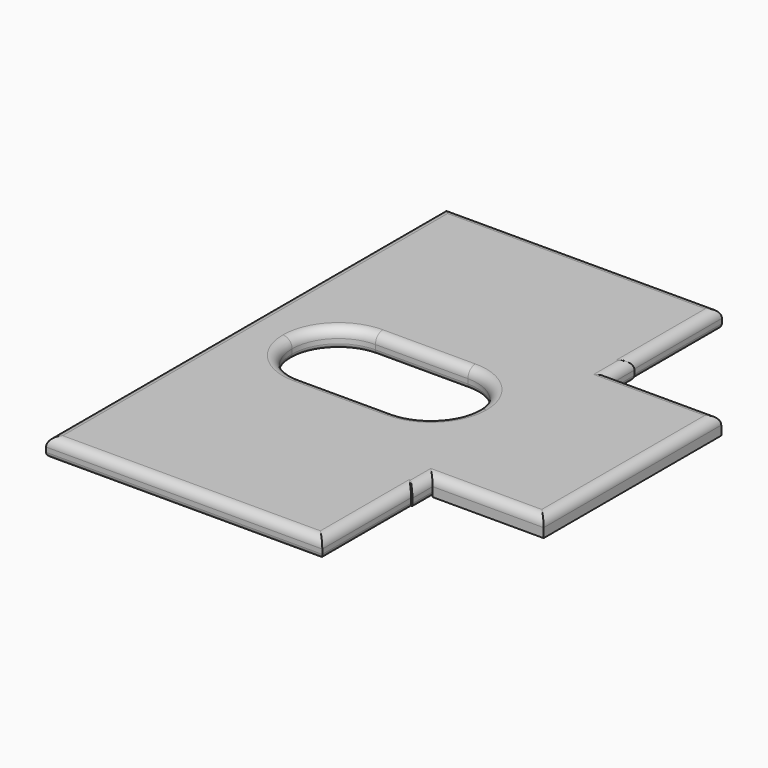
from build123d import *

# Parameters (mm, degrees)
F0_W     = 14.9271550402
F0_H     = 6
F1_DEPTH = 1
F2_R     = 0.25
F3_DEPTH = 1
F0_W_2   = 6
F0_H_2   = 12
F4_DEPTH = 1
F5_R     = 0.5


# Not quite as in the source:
# - a feature names something its author has since deleted; it is built from what else it names


with BuildPart() as f1:
    # F0 (on Top) → F1 (new body)
    with BuildSketch(Plane.XY):
        with Locations((-0.0364224799, 10.5)):
            Rectangle(F0_W, F0_H)
        Polygon((7.4271550402, 7.5), (-7.5, 7.5), (-7.5, -7.5), (7.4271550402, -7.5), (7.5, -7.5), (7.5, -6.1350027099), (7.5, 5.8649972901), (7.5, 7.5), align=None)
        with BuildLine():
            ThreePointArc((-5, 0), (-4.267766953, 1.767766953), (-2.5, 2.5))
            Line((-2.5, 2.5), (2.5, 2.5))
            ThreePointArc((2.5, 2.5), (4.267766953, 1.767766953), (5, 0))
            ThreePointArc((5, 0), (4.267766953, -1.767766953), (2.5, -2.5))
            Line((2.5, -2.5), (-2.5, -2.5))
            ThreePointArc((-2.5, -2.5), (-4.267766953, -1.767766953), (-5, 0))
        make_face(mode=Mode.SUBTRACT)
        with Locations((-0.0364224799, -10.5)):
            Rectangle(F0_W, F0_H)
    extrude(amount=F1_DEPTH)

    # F2
    f2_edges = [f1.edges().sort_by_distance(p)[0] for p in [
        (-0.036422, 13.5, 0),
        (-7.5, 0, 0),
        (-0.036422, -13.5, 0),
        (7.427155, -10.5, 0),
        (7.463578, -7.5, 0),
        (7.5, 0, 0),
        (7.463578, 7.5, 0),
        (7.427155, 10.5, 0),
        (-5, 0, 0),
        (0, 2.5, 0),
        (5, 0, 0),
        (0, -2.5, 0),
    ]]
    fillet(f2_edges, radius=F2_R)

    # F0 (on Top) → F3 (cut)
    with BuildSketch(Plane.XY):
        with BuildLine():
            Line((2.5, 2.5), (-2.5, 2.5))
            ThreePointArc((-2.5, 2.5), (-4.267766953, 1.767766953), (-5, 0))
            ThreePointArc((-5, 0), (-4.267766953, -1.767766953), (-2.5, -2.5))
            Line((-2.5, -2.5), (2.5, -2.5))
            ThreePointArc((2.5, -2.5), (4.267766953, -1.767766953), (5, 0))
            ThreePointArc((5, 0), (4.267766953, 1.767766953), (2.5, 2.5))
        make_face()
    extrude(amount=F3_DEPTH, mode=Mode.SUBTRACT)

    # F0 (on Top) → F4 (join)
    with BuildSketch(Plane.XY):
        with Locations((10.5, -0.1350027099)):
            Rectangle(F0_W_2, F0_H_2)
    extrude(amount=F4_DEPTH)

    # F5
    f5_edges = [f1.edges().sort_by_distance(p)[0] for p in [
        (-0.036422, 13.5, 1),
        (-7.5, 0, 1),
        (-0.036422, -13.5, 1),
        (7.427155, -10.5, 1),
        (7.463578, -7.5, 1),
        (7.5, -6.817501, 1),
        (10.5, -6.135003, 1),
        (13.5, -0.135003, 1),
        (10.5, 5.864997, 1),
        (7.5, 6.682499, 1),
        (7.463578, 7.5, 1),
        (7.427155, 10.5, 1),
        (-5, 0, 1),
        (0, 2.5, 1),
        (5, 0, 1),
        (0, -2.5, 1),
    ]]
    fillet(f5_edges, radius=F5_R)


solid = f1.part
